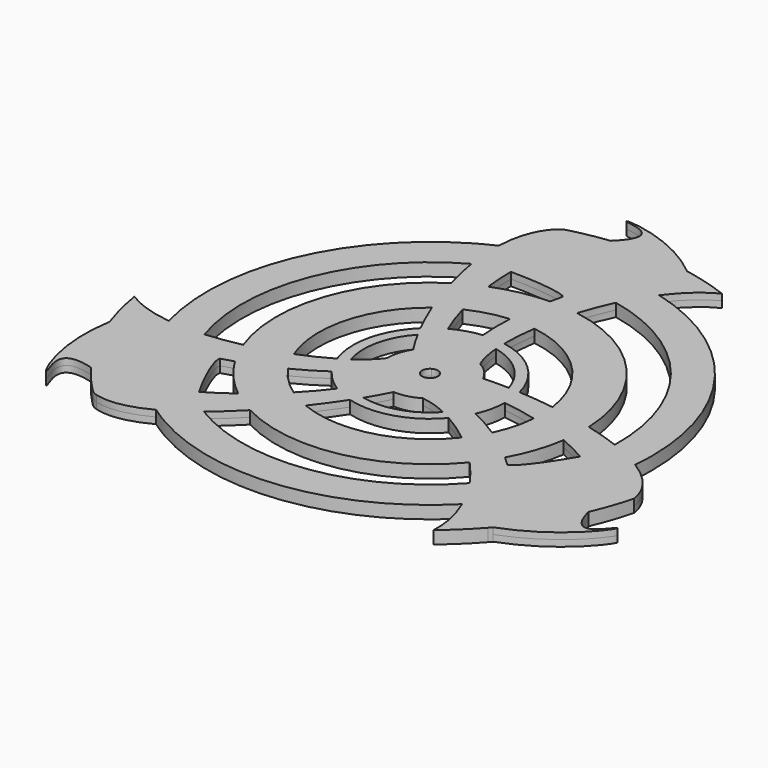
from build123d import *

# Parameters (mm, degrees)
F0_R     = 2.3749
F1_DEPTH = 1.905
F2_COUNT = 3
F3_R     = 5.08


# Not quite as in the source:
# - a feature names something its author has since deleted; it is built from what else it names


with BuildPart() as f1:
    # F0 (on Top) → F1 (new body, symmetric)
    with BuildSketch(Plane.XY):
        with BuildLine():
            ThreePointArc((-9.528872644, 17.3861879456), (-12.1755023676, 15.6472389654), (-14.5114994496, 13.5090831988))
            add(Edge.make_bspline(
                [(-10.6110147807, 6.9782781059), (-11.8921280006, 8.897792987), (-13.2068281317, 11.0978958561), (-14.5114994496, 13.5090831988)],
                knots=[0, 0, 0, 0, 7.786603859, 7.786603859, 7.786603859, 7.786603859], degree=3))
            ThreePointArc((-10.6110147807, 6.9782781059), (-8.5295013565, 9.4094424175), (-5.9062935719, 11.2430287842))
            add(Edge.make_bspline(
                [(-5.9062935719, 11.2430287842), (-7.1619609256, 12.9834047155), (-8.3819608859, 15.0567262616), (-9.528872644, 17.3861879456)],
                knots=[0, 0, 0, 0, 8.2558127914, 8.2558127914, 8.2558127914, 8.2558127914], degree=3))
        make_face()
        with BuildLine():
            ThreePointArc((-14.1894324685, 18.125199524), (-15.1485765447, 17.331574661), (-16.0634124943, 16.4872566123))
            add(Edge.make_bspline(
                [(-14.5114994496, 13.5090831988), (-15.0313153427, 14.4697646248), (-15.5495392236, 15.4639544104), (-16.0634124943, 16.4872566123)],
                knots=[7.786603859, 7.786603859, 7.786603859, 7.786603859, 10.8889947709, 10.8889947709, 10.8889947709, 10.8889947709], degree=3))
            ThreePointArc((-14.5114994496, 13.5090831988), (-12.1755023676, 15.6472389654), (-9.528872644, 17.3861879456))
            add(Edge.make_bspline(
                [(-9.528872644, 17.3861879456), (-9.8345228396, 18.0069858528), (-10.1349822073, 18.6459751962), (-10.4295424799, 19.3017022708)],
                knots=[8.2558127914, 8.2558127914, 8.2558127914, 8.2558127914, 10.4559740298, 10.4559740298, 10.4559740298, 10.4559740298], degree=3))
            add(Edge.make_bspline(
                [(-10.4295424842, 19.3017022678), (-11.6022425813, 19.0466590234), (-12.860295893, 18.6657552279), (-14.1894324685, 18.125199524)],
                knots=[9.5916797574, 9.5916797574, 9.5916797574, 9.5916797574, 12.336643885, 12.336643885, 12.336643885, 12.336643885], degree=3))
        make_face()
        with BuildLine():
            ThreePointArc((-14.2913508532, 30.1188677915), (-17.4869107202, 28.3830382397), (-20.4743892657, 26.3094714969))
            add(Edge.make_bspline(
                [(-16.0634124943, 16.4872566123), (-17.5969200818, 19.5410089294), (-19.0916831767, 22.8540227617), (-20.4743892657, 26.3094714969)],
                knots=[10.8889947709, 10.8889947709, 10.8889947709, 10.8889947709, 20.1471918293, 20.1471918293, 20.1471918293, 20.1471918293], degree=3))
            ThreePointArc((-16.0634124943, 16.4872566123), (-15.1485765447, 17.331574661), (-14.1894324685, 18.125199524))
            ThreePointArc((-14.1894324685, 18.125199524), (-12.5740143774, 19.2810013744), (-10.8649679271, 20.2932334414))
            add(Edge.make_bspline(
                [(-10.8649679271, 20.2932334414), (-12.1526094438, 23.2925410437), (-13.3157250851, 26.610829951), (-14.2913508532, 30.1188677915)],
                knots=[11.5512193248, 11.5512193248, 11.5512193248, 11.5512193248, 21.3706478137, 21.3706478137, 21.3706478137, 21.3706478137], degree=3))
        make_face()
        with BuildLine():
            ThreePointArc((-16.8266851474, 42.8522353349), (-20.8838064554, 41.0282589709), (-24.7459572878, 38.8212442377))
            add(Edge.make_bspline(
                [(-20.4743892657, 26.3094714969), (-22.090291021, 30.3476873699), (-23.5531512922, 34.5804332391), (-24.7459572878, 38.8212442377)],
                knots=[20.1471918293, 20.1471918293, 20.1471918293, 20.1471918293, 30.9667991167, 30.9667991167, 30.9667991167, 30.9667991167], degree=3))
            ThreePointArc((-20.4743892657, 26.3094714969), (-17.4869107202, 28.3830382397), (-14.2913508532, 30.1188677915))
            add(Edge.make_bspline(
                [(-14.2913508532, 30.1188677915), (-15.4197279706, 34.1761505693), (-16.2973095348, 38.4872507284), (-16.8266851474, 42.8522353349)],
                knots=[21.3706478137, 21.3706478137, 21.3706478137, 21.3706478137, 32.7274802957, 32.7274802957, 32.7274802957, 32.7274802957], degree=3))
        make_face()
        with BuildLine():
            ThreePointArc((-22.0791081901, 51.851132057), (-24.6247227209, 50.6917147567), (-27.1096722353, 49.4074142752))
            add(Edge.make_bspline(
                [(-24.7459572878, 38.8212442377), (-25.7472173213, 42.381047406), (-26.558192075, 45.946533415), (-27.1096722353, 49.4074142752)],
                knots=[30.9667991167, 30.9667991167, 30.9667991167, 30.9667991167, 40.0489469217, 40.0489469217, 40.0489469217, 40.0489469217], degree=3))
            ThreePointArc((-24.7459572878, 38.8212442377), (-20.8838064554, 41.0282589709), (-16.8266851474, 42.8522353349))
            add(Edge.make_bspline(
                [(-16.8266851474, 42.8522353349), (-17.1969594422, 45.9053446174), (-17.3968785128, 48.9848161636), (-17.3931086058, 52.0222330976)],
                knots=[32.7274802957, 32.7274802957, 32.7274802957, 32.7274802957, 40.6710708914, 40.6710708914, 40.6710708914, 40.6710708914], degree=3))
            add(Edge.make_bspline(
                [(-17.3931086058, 52.0222330976), (-19.1262917466, 52.0176549886), (-20.7372371311, 51.9617830814), (-22.0791081901, 51.851132057)],
                knots=[17.8698164727, 17.8698164727, 17.8698164727, 17.8698164727, 22.1848617745, 22.1848617745, 22.1848617745, 22.1848617745], degree=3))
        make_face()
        with BuildLine():
            ThreePointArc((-15.9984575055, 64.7271579976), (-22.0407399455, 62.926635121), (-27.8859395361, 60.5634378251))
            add(Edge.make_bspline(
                [(-27.1096722353, 49.4074142752), (-27.7318602874, 53.3120311158), (-28.0237458388, 57.083499355), (-27.8859395361, 60.5634378251)],
                knots=[40.0489469217, 40.0489469217, 40.0489469217, 40.0489469217, 50.2955600532, 50.2955600532, 50.2955600532, 50.2955600532], degree=3))
            ThreePointArc((-27.1096722353, 49.4074142752), (-24.6247227209, 50.6917147567), (-22.0791081901, 51.851132057))
            ThreePointArc((-22.0791081901, 51.851132057), (-19.7453181215, 52.7839874047), (-17.3722566192, 53.6118607588))
            add(Edge.make_bspline(
                [(-17.3722566192, 53.6118607588), (-17.2756028467, 57.4510532594), (-16.8404836195, 61.2029772384), (-15.9984575055, 64.7271579976)],
                knots=[42.0605104223, 42.0605104223, 42.0605104223, 42.0605104223, 52.1568002558, 52.1568002558, 52.1568002558, 52.1568002558], degree=3))
        make_face()
        with BuildLine():
            ThreePointArc((-8.9715342618, 78.866356566), (-15.2520877956, 77.8958563909), (-21.4348712844, 76.4260225187))
            add(Edge.make_bspline(
                [(-27.8859395361, 60.5634378251), (-27.6170866573, 67.3526155134), (-25.7127420915, 73.0321735767), (-21.4348712844, 76.4260225187)],
                knots=[50.2955600532, 50.2955600532, 50.2955600532, 50.2955600532, 70.286165592, 70.286165592, 70.286165592, 70.286165592], degree=3))
            ThreePointArc((-27.8859395361, 60.5634378251), (-22.0407399455, 62.926635121), (-15.9984575055, 64.7271579976))
            add(Edge.make_bspline(
                [(-15.9984575055, 64.7271579976), (-14.7027650739, 70.1500947234), (-12.4435814186, 75.0337714842), (-8.9715342618, 78.866356566)],
                knots=[52.1568002558, 52.1568002558, 52.1568002558, 52.1568002558, 67.6927629867, 67.6927629867, 67.6927629867, 67.6927629867], degree=3))
        make_face()
        with BuildLine():
            ThreePointArc((12.7, 0), (10.9401596307, 6.4500315701), (6.1483610621, 11.1125))
            ThreePointArc((6.1483610621, 11.1125), (3.175, 12.2967221242), (0, 12.7))
            ThreePointArc((0, 12.7), (-3.0416717805, 12.3303784524), (-5.9062935719, 11.2430287842))
            ThreePointArc((-5.9062935719, 11.2430287842), (-8.5295013565, 9.4094424175), (-10.6110147807, 6.9782781059))
            ThreePointArc((-10.6110147807, 6.9782781059), (-3.6421224777, -12.1665502036), (12.7, 0))
        make_face()
        Circle(F0_R, mode=Mode.SUBTRACT)
        with BuildLine():
            add(Edge.make_bspline(
                [(14.6249362914, 78.016035938), (0, 90.1043615439), (-24.9924816186, 89.1573770228), (0, 87.6129916924), (-8.9715342618, 78.866356566)],
                knots=[0, 0, 0, 0, 0.6253977609, 1, 1, 1, 1], degree=3))
            ThreePointArc((-8.9715342618, 78.866356566), (2.858496094, 79.3235124353), (14.6249362914, 78.016035938))
        make_face()
        with BuildLine():
            add(Edge.make_bspline(
                [(6.3746301433, 66.3695691981), (9.0305383212, 71.2117016577), (12.2180589412, 75.2172352435), (15.8720328719, 77.7719049369)],
                knots=[51.5599598573, 51.5599598573, 51.5599598573, 51.5599598573, 66.9796554157, 66.9796554157, 66.9796554157, 66.9796554157], degree=3))
            ThreePointArc((15.8720328719, 77.7719049369), (15.2489731465, 77.8964661777), (14.6249362914, 78.016035938))
            ThreePointArc((14.6249362914, 78.016035938), (2.858496094, 79.3235124353), (-8.9715342618, 78.866356566))
            add(Edge.make_bspline(
                [(-15.9984575055, 64.7271579976), (-14.7027650739, 70.1500947234), (-12.4435814186, 75.0337714842), (-8.9715342618, 78.866356566)],
                knots=[52.1568002558, 52.1568002558, 52.1568002558, 52.1568002558, 67.6927629867, 67.6927629867, 67.6927629867, 67.6927629867], degree=3))
            ThreePointArc((-15.9984575055, 64.7271579976), (-4.8814846012, 66.4960655459), (6.3746301433, 66.3695691981))
        make_face()
        with BuildLine():
            add(Edge.make_bspline(
                [(17.1146888189, 64.4410044276), (20.2336975007, 68.6370859266), (23.89394856, 72.0708190073), (28.0724925102, 74.2450388192)],
                knots=[52.8219144622, 52.8219144622, 52.8219144622, 52.8219144622, 66.8310182289, 66.8310182289, 66.8310182289, 66.8310182289], degree=3))
            ThreePointArc((28.0724925102, 74.2450388192), (22.0429132357, 76.2528727399), (15.8720328719, 77.7719049369))
            add(Edge.make_bspline(
                [(6.3746301433, 66.3695691981), (9.0305383212, 71.2117016577), (12.2180589412, 75.2172352435), (15.8720328719, 77.7719049369)],
                knots=[51.5599598573, 51.5599598573, 51.5599598573, 51.5599598573, 66.9796554157, 66.9796554157, 66.9796554157, 66.9796554157], degree=3))
            ThreePointArc((6.3746301433, 66.3695691981), (11.7841786666, 65.6253667278), (17.1146888189, 64.4410044276))
        make_face()
        with BuildLine():
            add(Edge.make_bspline(
                [(7.7682782444, 45.3773650554), (8.8202491469, 48.7226402164), (10.0965565472, 52.0214234611), (11.5915484463, 55.1512730468)],
                knots=[34.6747463877, 34.6747463877, 34.6747463877, 34.6747463877, 43.4559365162, 43.4559365162, 43.4559365162, 43.4559365162], degree=3))
            ThreePointArc((11.5915484463, 55.1512730468), (6.8136819177, 55.942833793), (1.9854971672, 56.3212634363))
            add(Edge.make_bspline(
                [(0, 49.6875531971), (0.5760471795, 51.9412030755), (1.2390854665, 54.1638080047), (1.9854971672, 56.3212634363)],
                knots=[35.9138489532, 35.9138489532, 35.9138489532, 35.9138489532, 41.7963404213, 41.7963404213, 41.7963404213, 41.7963404213], degree=3))
            add(Edge.make_bspline(
                [(-0.8534126769, 46.0295893209), (-0.5944813694, 47.2543537136), (-0.3098228581, 48.4754437182), (0, 49.6875531971)],
                knots=[32.7499929625, 32.7499929625, 32.7499929625, 32.7499929625, 35.9138489532, 35.9138489532, 35.9138489532, 35.9138489532], degree=3))
            ThreePointArc((-0.8534126769, 46.0295893209), (3.4727785097, 45.9063308888), (7.7682782444, 45.3773650554))
        make_face()
        with BuildLine():
            add(Edge.make_bspline(
                [(4.9039542617, 32.9748409981), (5.5079423386, 37.0254762013), (6.4662888393, 41.2370292282), (7.7682782444, 45.3773650554)],
                knots=[23.8065593645, 23.8065593645, 23.8065593645, 23.8065593645, 34.6747463877, 34.6747463877, 34.6747463877, 34.6747463877], degree=3))
            ThreePointArc((7.7682782444, 45.3773650554), (3.4727785097, 45.9063308888), (-0.8534126769, 46.0295893209))
            add(Edge.make_bspline(
                [(-2.604181902, 33.2356306224), (-2.3532796725, 37.3928516921), (-1.7615944725, 41.7338217054), (-0.8534126769, 46.0295893209)],
                knots=[21.6530095861, 21.6530095861, 21.6530095861, 21.6530095861, 32.7499929625, 32.7499929625, 32.7499929625, 32.7499929625], degree=3))
            ThreePointArc((-2.604181902, 33.2356306224), (1.1572558203, 33.3174078406), (4.9039542617, 32.9748409981))
        make_face()
        with BuildLine():
            add(Edge.make_bspline(
                [(6.1483610621, 11.1125), (5.1712773611, 13.2934923084), (4.555008051, 16.1137421587), (4.2895532846, 19.3566184486)],
                knots=[0, 0, 0, 0, 10.6206349908, 10.6206349908, 10.6206349908, 10.6206349908], degree=3))
            ThreePointArc((4.2895532846, 19.3566184486), (1.1399558403, 19.7934192556), (-2.0389634971, 19.7210946198))
            add(Edge.make_bspline(
                [(-1.8716278865, 18.8067218094), (-1.9304421703, 19.1076938448), (-1.9862147094, 19.4125413232), (-2.0389634971, 19.7210946198)],
                knots=[7.6177317002, 7.6177317002, 7.6177317002, 7.6177317002, 8.6218547112, 8.6218547112, 8.6218547112, 8.6218547112], degree=3))
            add(Edge.make_bspline(
                [(0, 12.7), (-0.8041789521, 14.4631498702), (-1.4254361064, 16.5234117066), (-1.8716278865, 18.8067218094)],
                knots=[0, 0, 0, 0, 7.6177317002, 7.6177317002, 7.6177317002, 7.6177317002], degree=3))
            ThreePointArc((0, 12.7), (3.175, 12.2967221242), (6.1483610621, 11.1125))
        make_face()
        with BuildLine():
            add(Edge.make_bspline(
                [(-2.604181902, 33.2356306224), (-2.3532796725, 37.3928516921), (-1.7615944725, 41.7338217054), (-0.8534126769, 46.0295893209)],
                knots=[21.6530095861, 21.6530095861, 21.6530095861, 21.6530095861, 32.7499929625, 32.7499929625, 32.7499929625, 32.7499929625], degree=3))
            ThreePointArc((-0.8534126769, 46.0295893209), (-8.9816679607, 45.1528631085), (-16.8266851474, 42.8522353349))
            add(Edge.make_bspline(
                [(-14.2913508532, 30.1188677915), (-15.4197279706, 34.1761505693), (-16.2973095348, 38.4872507284), (-16.8266851474, 42.8522353349)],
                knots=[21.3706478137, 21.3706478137, 21.3706478137, 21.3706478137, 32.7274802957, 32.7274802957, 32.7274802957, 32.7274802957], degree=3))
            ThreePointArc((-14.2913508532, 30.1188677915), (-8.5903032197, 32.2117307334), (-2.604181902, 33.2356306224))
        make_face()
        with BuildLine():
            ThreePointArc((-22.0791081901, 51.851132057), (-24.6247227209, 50.6917147567), (-27.1096722353, 49.4074142752))
            add(Edge.make_bspline(
                [(-24.7459572878, 38.8212442377), (-25.7472173213, 42.381047406), (-26.558192075, 45.946533415), (-27.1096722353, 49.4074142752)],
                knots=[30.9667991167, 30.9667991167, 30.9667991167, 30.9667991167, 40.0489469217, 40.0489469217, 40.0489469217, 40.0489469217], degree=3))
            ThreePointArc((-24.7459572878, 38.8212442377), (-20.8838064554, 41.0282589709), (-16.8266851474, 42.8522353349))
            add(Edge.make_bspline(
                [(-16.8266851474, 42.8522353349), (-17.1969594422, 45.9053446174), (-17.3968785128, 48.9848161636), (-17.3931086058, 52.0222330976)],
                knots=[32.7274802957, 32.7274802957, 32.7274802957, 32.7274802957, 40.6710708914, 40.6710708914, 40.6710708914, 40.6710708914], degree=3))
            add(Edge.make_bspline(
                [(-17.3931086058, 52.0222330976), (-19.1262917466, 52.0176549886), (-20.7372371311, 51.9617830814), (-22.0791081901, 51.851132057)],
                knots=[17.8698164727, 17.8698164727, 17.8698164727, 17.8698164727, 22.1848617745, 22.1848617745, 22.1848617745, 22.1848617745], degree=3))
        make_face()
        with BuildLine():
            add(Edge.make_bspline(
                [(11.5915484463, 55.1512730468), (13.1861000905, 58.4895565556), (15.0294329015, 61.6356567455), (17.1146888189, 64.4410044276)],
                knots=[43.4559365162, 43.4559365162, 43.4559365162, 43.4559365162, 52.8219144622, 52.8219144622, 52.8219144622, 52.8219144622], degree=3))
            ThreePointArc((17.1146888189, 64.4410044276), (11.7841786666, 65.6253667278), (6.3746301433, 66.3695691981))
            add(Edge.make_bspline(
                [(1.9854971672, 56.3212634363), (3.2243735562, 59.902156651), (4.6929317851, 63.3035723102), (6.3746301433, 66.3695691981)],
                knots=[41.7963404213, 41.7963404213, 41.7963404213, 41.7963404213, 51.5599598573, 51.5599598573, 51.5599598573, 51.5599598573], degree=3))
            ThreePointArc((1.9854971672, 56.3212634363), (6.8136819177, 55.942833793), (11.5915484463, 55.1512730468))
        make_face()
        with BuildLine():
            add(Edge.make_bspline(
                [(0, 49.6875531971), (0.5760471795, 51.9412030755), (1.2390854665, 54.1638080047), (1.9854971672, 56.3212634363)],
                knots=[35.9138489532, 35.9138489532, 35.9138489532, 35.9138489532, 41.7963404213, 41.7963404213, 41.7963404213, 41.7963404213], degree=3))
            ThreePointArc((1.9854971672, 56.3212634363), (-7.811741632, 55.8122173609), (-17.3722566192, 53.6118607588))
            add(Edge.make_bspline(
                [(-17.3931086058, 52.0222330976), (-17.392449199, 52.5535176734), (-17.3855579977, 53.0835156028), (-17.3722566192, 53.6118607588)],
                knots=[40.6710708914, 40.6710708914, 40.6710708914, 40.6710708914, 42.0605104223, 42.0605104223, 42.0605104223, 42.0605104223], degree=3))
            add(Edge.make_bspline(
                [(0, 49.6875531971), (-0.9415073978, 51.1804521144), (-10.2155096531, 52.041192335), (-17.3931086058, 52.0222330976)],
                knots=[0, 0, 0, 0, 17.8698164727, 17.8698164727, 17.8698164727, 17.8698164727], degree=3))
        make_face()
        with BuildLine():
            add(Edge.make_bspline(
                [(-17.3931086058, 52.0222330976), (-17.392449199, 52.5535176734), (-17.3855579977, 53.0835156028), (-17.3722566192, 53.6118607588)],
                knots=[40.6710708914, 40.6710708914, 40.6710708914, 40.6710708914, 42.0605104223, 42.0605104223, 42.0605104223, 42.0605104223], degree=3))
            ThreePointArc((-17.3722566192, 53.6118607588), (-19.7453181215, 52.7839874047), (-22.0791081901, 51.851132057))
            add(Edge.make_bspline(
                [(-17.3931086058, 52.0222330976), (-19.1262917466, 52.0176549886), (-20.7372371311, 51.9617830814), (-22.0791081901, 51.851132057)],
                knots=[17.8698164727, 17.8698164727, 17.8698164727, 17.8698164727, 22.1848617745, 22.1848617745, 22.1848617745, 22.1848617745], degree=3))
        make_face()
        with BuildLine():
            ThreePointArc((-9.528872644, 17.3861879456), (-12.1755023676, 15.6472389654), (-14.5114994496, 13.5090831988))
            add(Edge.make_bspline(
                [(-10.6110147807, 6.9782781059), (-11.8921280006, 8.897792987), (-13.2068281317, 11.0978958561), (-14.5114994496, 13.5090831988)],
                knots=[0, 0, 0, 0, 7.786603859, 7.786603859, 7.786603859, 7.786603859], degree=3))
            ThreePointArc((-10.6110147807, 6.9782781059), (-8.5295013565, 9.4094424175), (-5.9062935719, 11.2430287842))
            add(Edge.make_bspline(
                [(-5.9062935719, 11.2430287842), (-7.1619609256, 12.9834047155), (-8.3819608859, 15.0567262616), (-9.528872644, 17.3861879456)],
                knots=[0, 0, 0, 0, 8.2558127914, 8.2558127914, 8.2558127914, 8.2558127914], degree=3))
        make_face()
        with BuildLine():
            add(Edge.make_bspline(
                [(4.1415758337, 22.6431049367), (4.1061899388, 25.8466221872), (4.3628839221, 29.346162471), (4.9039542617, 32.9748409981)],
                knots=[14.0705167684, 14.0705167684, 14.0705167684, 14.0705167684, 23.8065593645, 23.8065593645, 23.8065593645, 23.8065593645], degree=3))
            ThreePointArc((4.9039542617, 32.9748409981), (1.1572558203, 33.3174078406), (-2.604181902, 33.2356306224))
            add(Edge.make_bspline(
                [(-2.4626280821, 22.8866405244), (-2.7822475772, 26.0926504323), (-2.8239889999, 29.5936275198), (-2.604181902, 33.2356306224)],
                knots=[11.9313115552, 11.9313115552, 11.9313115552, 11.9313115552, 21.6530095861, 21.6530095861, 21.6530095861, 21.6530095861], degree=3))
            ThreePointArc((-2.4626280821, 22.8866405244), (0.8482592668, 23.0031151755), (4.1415758337, 22.6431049367))
        make_face()
        with BuildLine():
            add(Edge.make_bspline(
                [(-1.8716278865, 18.8067218094), (-1.9304421703, 19.1076938448), (-1.9862147094, 19.4125413232), (-2.0389634971, 19.7210946198)],
                knots=[7.6177317002, 7.6177317002, 7.6177317002, 7.6177317002, 8.6218547112, 8.6218547112, 8.6218547112, 8.6218547112], degree=3))
            ThreePointArc((-2.0389634971, 19.7210946198), (-2.9190249054, 19.6101565202), (-3.7932433816, 19.4599653081))
            add(Edge.make_bspline(
                [(-1.8716278865, 18.8067218094), (-2.3377563596, 19.0525011146), (-2.9857121543, 19.2878131642), (-3.7932433816, 19.4599653081)],
                knots=[0, 0, 0, 0, 3.1831087405, 3.1831087405, 3.1831087405, 3.1831087405], degree=3))
        make_face()
        with BuildLine():
            add(Edge.make_bspline(
                [(-2.0389634971, 19.7210946198), (-2.2128165356, 20.7380455391), (-2.3538233319, 21.7952518186), (-2.4626280821, 22.8866405244)],
                knots=[8.6218547112, 8.6218547112, 8.6218547112, 8.6218547112, 11.9313115552, 11.9313115552, 11.9313115552, 11.9313115552], degree=3))
            ThreePointArc((-2.4626280821, 22.8866405244), (-6.788788104, 21.9948904894), (-10.8649679271, 20.2932334414))
            add(Edge.make_bspline(
                [(-10.4295424799, 19.3017022708), (-10.5761752571, 19.6281247079), (-10.7213461965, 19.9586948739), (-10.8649679271, 20.2932334414)],
                knots=[10.4559740298, 10.4559740298, 10.4559740298, 10.4559740298, 11.5512193248, 11.5512193248, 11.5512193248, 11.5512193248], degree=3))
            add(Edge.make_bspline(
                [(-3.7932433816, 19.4599653081), (-5.4190506161, 19.8065602032), (-7.6916808932, 19.8971427426), (-10.4295424842, 19.3017022678)],
                knots=[3.1831087405, 3.1831087405, 3.1831087405, 3.1831087405, 9.5916797574, 9.5916797574, 9.5916797574, 9.5916797574], degree=3))
            ThreePointArc((-3.7932433816, 19.4599653081), (-2.9190249054, 19.6101565202), (-2.0389634971, 19.7210946198))
        make_face()
        with BuildLine():
            ThreePointArc((-10.8649679271, 20.2932334414), (-12.5740143774, 19.2810013744), (-14.1894324685, 18.125199524))
            add(Edge.make_bspline(
                [(-10.4295424842, 19.3017022678), (-11.6022425813, 19.0466590234), (-12.860295893, 18.6657552279), (-14.1894324685, 18.125199524)],
                knots=[9.5916797574, 9.5916797574, 9.5916797574, 9.5916797574, 12.336643885, 12.336643885, 12.336643885, 12.336643885], degree=3))
            add(Edge.make_bspline(
                [(-10.4295424799, 19.3017022708), (-10.5761752571, 19.6281247079), (-10.7213461965, 19.9586948739), (-10.8649679271, 20.2932334414)],
                knots=[10.4559740298, 10.4559740298, 10.4559740298, 10.4559740298, 11.5512193248, 11.5512193248, 11.5512193248, 11.5512193248], degree=3))
        make_face()
        with BuildLine():
            ThreePointArc((-14.2913508532, 30.1188677915), (-17.4869107202, 28.3830382397), (-20.4743892657, 26.3094714969))
            add(Edge.make_bspline(
                [(-16.0634124943, 16.4872566123), (-17.5969200818, 19.5410089294), (-19.0916831767, 22.8540227617), (-20.4743892657, 26.3094714969)],
                knots=[10.8889947709, 10.8889947709, 10.8889947709, 10.8889947709, 20.1471918293, 20.1471918293, 20.1471918293, 20.1471918293], degree=3))
            ThreePointArc((-16.0634124943, 16.4872566123), (-15.1485765447, 17.331574661), (-14.1894324685, 18.125199524))
            ThreePointArc((-14.1894324685, 18.125199524), (-12.5740143774, 19.2810013744), (-10.8649679271, 20.2932334414))
            add(Edge.make_bspline(
                [(-10.8649679271, 20.2932334414), (-12.1526094438, 23.2925410437), (-13.3157250851, 26.610829951), (-14.2913508532, 30.1188677915)],
                knots=[11.5512193248, 11.5512193248, 11.5512193248, 11.5512193248, 21.3706478137, 21.3706478137, 21.3706478137, 21.3706478137], degree=3))
        make_face()
        with BuildLine():
            add(Edge.make_bspline(
                [(-2.0389634971, 19.7210946198), (-2.2128165356, 20.7380455391), (-2.3538233319, 21.7952518186), (-2.4626280821, 22.8866405244)],
                knots=[8.6218547112, 8.6218547112, 8.6218547112, 8.6218547112, 11.9313115552, 11.9313115552, 11.9313115552, 11.9313115552], degree=3))
            ThreePointArc((-2.4626280821, 22.8866405244), (-6.788788104, 21.9948904894), (-10.8649679271, 20.2932334414))
            add(Edge.make_bspline(
                [(-10.4295424799, 19.3017022708), (-10.5761752571, 19.6281247079), (-10.7213461965, 19.9586948739), (-10.8649679271, 20.2932334414)],
                knots=[10.4559740298, 10.4559740298, 10.4559740298, 10.4559740298, 11.5512193248, 11.5512193248, 11.5512193248, 11.5512193248], degree=3))
            add(Edge.make_bspline(
                [(-3.7932433816, 19.4599653081), (-5.4190506161, 19.8065602032), (-7.6916808932, 19.8971427426), (-10.4295424842, 19.3017022678)],
                knots=[3.1831087405, 3.1831087405, 3.1831087405, 3.1831087405, 9.5916797574, 9.5916797574, 9.5916797574, 9.5916797574], degree=3))
            ThreePointArc((-3.7932433816, 19.4599653081), (-2.9190249054, 19.6101565202), (-2.0389634971, 19.7210946198))
        make_face()
        with BuildLine():
            ThreePointArc((-3.7932433816, 19.4599653081), (-6.7412782161, 18.6449487304), (-9.528872644, 17.3861879456))
            add(Edge.make_bspline(
                [(-5.9062935719, 11.2430287842), (-7.1619609256, 12.9834047155), (-8.3819608859, 15.0567262616), (-9.528872644, 17.3861879456)],
                knots=[0, 0, 0, 0, 8.2558127914, 8.2558127914, 8.2558127914, 8.2558127914], degree=3))
            ThreePointArc((-5.9062935719, 11.2430287842), (-3.0416717805, 12.3303784524), (0, 12.7))
            add(Edge.make_bspline(
                [(0, 12.7), (-0.8041789521, 14.4631498702), (-1.4254361064, 16.5234117066), (-1.8716278865, 18.8067218094)],
                knots=[0, 0, 0, 0, 7.6177317002, 7.6177317002, 7.6177317002, 7.6177317002], degree=3))
            add(Edge.make_bspline(
                [(-1.8716278865, 18.8067218094), (-2.3377563596, 19.0525011146), (-2.9857121543, 19.2878131642), (-3.7932433816, 19.4599653081)],
                knots=[0, 0, 0, 0, 3.1831087405, 3.1831087405, 3.1831087405, 3.1831087405], degree=3))
        make_face()
        with BuildLine():
            add(Edge.make_bspline(
                [(4.2895532846, 19.3566184486), (4.2033260899, 20.409996126), (4.1541145169, 21.5079665396), (4.1415758337, 22.6431049367)],
                knots=[10.6206349908, 10.6206349908, 10.6206349908, 10.6206349908, 14.0705167684, 14.0705167684, 14.0705167684, 14.0705167684], degree=3))
            ThreePointArc((4.1415758337, 22.6431049367), (0.8482592668, 23.0031151755), (-2.4626280821, 22.8866405244))
            add(Edge.make_bspline(
                [(-2.0389634971, 19.7210946198), (-2.2128165356, 20.7380455391), (-2.3538233319, 21.7952518186), (-2.4626280821, 22.8866405244)],
                knots=[8.6218547112, 8.6218547112, 8.6218547112, 8.6218547112, 11.9313115552, 11.9313115552, 11.9313115552, 11.9313115552], degree=3))
            ThreePointArc((-2.0389634971, 19.7210946198), (1.1399558403, 19.7934192556), (4.2895532846, 19.3566184486))
        make_face()
        with BuildLine():
            ThreePointArc((-14.1894324685, 18.125199524), (-15.1485765447, 17.331574661), (-16.0634124943, 16.4872566123))
            add(Edge.make_bspline(
                [(-14.5114994496, 13.5090831988), (-15.0313153427, 14.4697646248), (-15.5495392236, 15.4639544104), (-16.0634124943, 16.4872566123)],
                knots=[7.786603859, 7.786603859, 7.786603859, 7.786603859, 10.8889947709, 10.8889947709, 10.8889947709, 10.8889947709], degree=3))
            ThreePointArc((-14.5114994496, 13.5090831988), (-12.1755023676, 15.6472389654), (-9.528872644, 17.3861879456))
            add(Edge.make_bspline(
                [(-9.528872644, 17.3861879456), (-9.8345228396, 18.0069858528), (-10.1349822073, 18.6459751962), (-10.4295424799, 19.3017022708)],
                knots=[8.2558127914, 8.2558127914, 8.2558127914, 8.2558127914, 10.4559740298, 10.4559740298, 10.4559740298, 10.4559740298], degree=3))
            add(Edge.make_bspline(
                [(-10.4295424842, 19.3017022678), (-11.6022425813, 19.0466590234), (-12.860295893, 18.6657552279), (-14.1894324685, 18.125199524)],
                knots=[9.5916797574, 9.5916797574, 9.5916797574, 9.5916797574, 12.336643885, 12.336643885, 12.336643885, 12.336643885], degree=3))
        make_face()
        with BuildLine():
            ThreePointArc((23.01875, 0), (17.6804517799, 14.7398940437), (4.1415758337, 22.6431049367))
            add(Edge.make_bspline(
                [(4.2895532846, 19.3566184486), (4.2033260899, 20.409996126), (4.1541145169, 21.5079665396), (4.1415758337, 22.6431049367)],
                knots=[10.6206349908, 10.6206349908, 10.6206349908, 10.6206349908, 14.0705167684, 14.0705167684, 14.0705167684, 14.0705167684], degree=3))
            ThreePointArc((4.2895532846, 19.3566184486), (15.461639085, 12.410344957), (19.8262186295, 0))
            ThreePointArc((19.8262186295, 0), (-7.2584703766, -18.4497575306), (-14.5114994496, 13.5090831988))
            add(Edge.make_bspline(
                [(-14.5114994496, 13.5090831988), (-15.0313153427, 14.4697646248), (-15.5495392236, 15.4639544104), (-16.0634124943, 16.4872566123)],
                knots=[7.786603859, 7.786603859, 7.786603859, 7.786603859, 10.8889947709, 10.8889947709, 10.8889947709, 10.8889947709], degree=3))
            ThreePointArc((-16.0634124943, 16.4872566123), (-8.94715528, -21.2087544179), (23.01875, 0))
        make_face()
        with BuildLine():
            ThreePointArc((46.0375, 0), (35.1929219867, 29.680122107), (7.7682782444, 45.3773650554))
            add(Edge.make_bspline(
                [(4.9039542617, 32.9748409981), (5.5079423386, 37.0254762013), (6.4662888393, 41.2370292282), (7.7682782444, 45.3773650554)],
                knots=[23.8065593645, 23.8065593645, 23.8065593645, 23.8065593645, 34.6747463877, 34.6747463877, 34.6747463877, 34.6747463877], degree=3))
            ThreePointArc((4.9039542617, 32.9748409981), (25.2475194965, 21.7704309908), (33.3375, 0))
            ThreePointArc((33.3375, 0), (-14.6428131536, -29.9495731054), (-20.4743892657, 26.3094714969))
            add(Edge.make_bspline(
                [(-20.4743892657, 26.3094714969), (-22.090291021, 30.3476873699), (-23.5531512922, 34.5804332391), (-24.7459572878, 38.8212442377)],
                knots=[20.1471918293, 20.1471918293, 20.1471918293, 20.1471918293, 30.9667991167, 30.9667991167, 30.9667991167, 30.9667991167], degree=3))
            ThreePointArc((-24.7459572878, 38.8212442377), (-22.1383083998, -40.3651670063), (46.0375, 0))
        make_face()
        with BuildLine():
            ThreePointArc((-15.9984575055, 64.7271579976), (-22.0407399455, 62.926635121), (-27.8859395361, 60.5634378251))
            add(Edge.make_bspline(
                [(-27.1096722353, 49.4074142752), (-27.7318602874, 53.3120311158), (-28.0237458388, 57.083499355), (-27.8859395361, 60.5634378251)],
                knots=[40.0489469217, 40.0489469217, 40.0489469217, 40.0489469217, 50.2955600532, 50.2955600532, 50.2955600532, 50.2955600532], degree=3))
            ThreePointArc((-27.1096722353, 49.4074142752), (-24.6247227209, 50.6917147567), (-22.0791081901, 51.851132057))
            ThreePointArc((-22.0791081901, 51.851132057), (-19.7453181215, 52.7839874047), (-17.3722566192, 53.6118607588))
            add(Edge.make_bspline(
                [(-17.3722566192, 53.6118607588), (-17.2756028467, 57.4510532594), (-16.8404836195, 61.2029772384), (-15.9984575055, 64.7271579976)],
                knots=[42.0605104223, 42.0605104223, 42.0605104223, 42.0605104223, 52.1568002558, 52.1568002558, 52.1568002558, 52.1568002558], degree=3))
        make_face()
        with BuildLine():
            add(Edge.make_bspline(
                [(0, 49.6875531971), (0.5760471795, 51.9412030755), (1.2390854665, 54.1638080047), (1.9854971672, 56.3212634363)],
                knots=[35.9138489532, 35.9138489532, 35.9138489532, 35.9138489532, 41.7963404213, 41.7963404213, 41.7963404213, 41.7963404213], degree=3))
            ThreePointArc((1.9854971672, 56.3212634363), (-7.811741632, 55.8122173609), (-17.3722566192, 53.6118607588))
            add(Edge.make_bspline(
                [(-17.3931086058, 52.0222330976), (-17.392449199, 52.5535176734), (-17.3855579977, 53.0835156028), (-17.3722566192, 53.6118607588)],
                knots=[40.6710708914, 40.6710708914, 40.6710708914, 40.6710708914, 42.0605104223, 42.0605104223, 42.0605104223, 42.0605104223], degree=3))
            add(Edge.make_bspline(
                [(0, 49.6875531971), (-0.9415073978, 51.1804521144), (-10.2155096531, 52.041192335), (-17.3931086058, 52.0222330976)],
                knots=[0, 0, 0, 0, 17.8698164727, 17.8698164727, 17.8698164727, 17.8698164727], degree=3))
        make_face()
        with BuildLine():
            ThreePointArc((66.675, 0), (52.8520458544, 40.6474706962), (17.1146888189, 64.4410044276))
            add(Edge.make_bspline(
                [(11.5915484463, 55.1512730468), (13.1861000905, 58.4895565556), (15.0294329015, 61.6356567455), (17.1146888189, 64.4410044276)],
                knots=[43.4559365162, 43.4559365162, 43.4559365162, 43.4559365162, 52.8219144622, 52.8219144622, 52.8219144622, 52.8219144622], degree=3))
            ThreePointArc((11.5915484463, 55.1512730468), (43.7566173064, 35.5159873292), (56.35625, 0))
            ThreePointArc((56.35625, 0), (-28.7073810034, -48.4965276075), (-27.1096722353, 49.4074142752))
            add(Edge.make_bspline(
                [(-27.1096722353, 49.4074142752), (-27.7318602874, 53.3120311158), (-28.0237458388, 57.083499355), (-27.8859395361, 60.5634378251)],
                knots=[40.0489469217, 40.0489469217, 40.0489469217, 40.0489469217, 50.2955600532, 50.2955600532, 50.2955600532, 50.2955600532], degree=3))
            ThreePointArc((-27.8859395361, 60.5634378251), (-35.9601210122, -56.146463128), (66.675, 0))
        make_face()
    extrude(amount=F1_DEPTH, both=True)

    # F2: F1 ×3 about axis
    f2_axis = Axis((0, 0, 1.905), (0, 0, 1))


with BuildPart() as f1_1:
    add(f1.part)
    for i in range(1, F2_COUNT):
        add(f1.part.rotate(f2_axis, i * 360 / F2_COUNT))

    # F3
    f3_edges = [f1_1.edges().sort_by_distance(p)[0] for p in [
        (-21.434871, 76.426023, 0.9525),
        (-21.434871, 76.426023, -0.9525),
        (-55.469441, -56.776154, -0.9525),
    ]]
    fillet(f3_edges, radius=F3_R)


solid = f1_1.part
